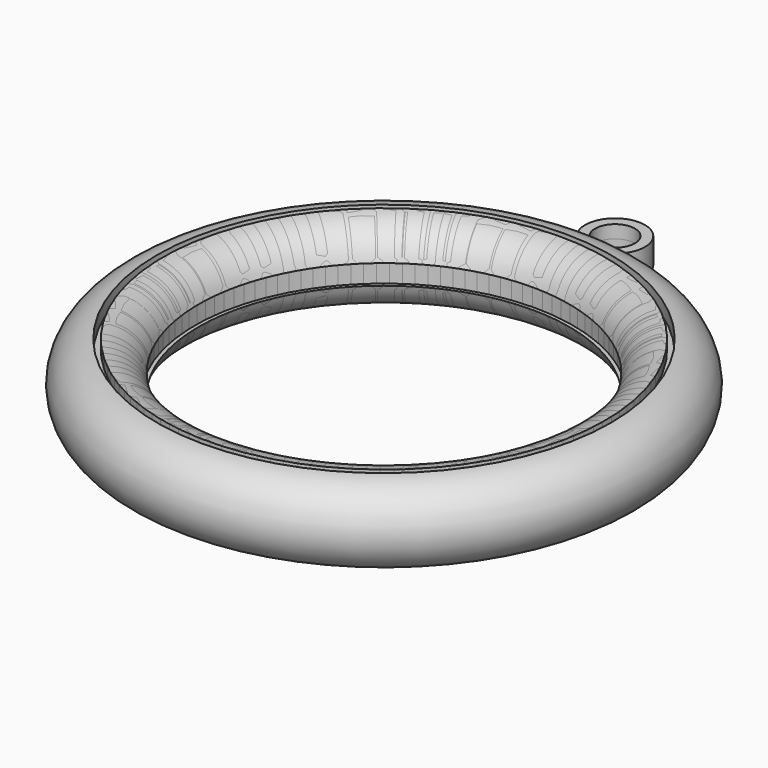
from build123d import *

# Parameters (mm, degrees)
F3_R          = 3
F3_R_2        = 2
F4_DEPTH      = 1.3
F4_DEPTH_BACK = 1.3
F1_R          = 1.5


with BuildPart() as f2:
    # F2: sweep along a path in F0
    with BuildLine(Plane.XY) as f2_path:
        CenterArc((0, 0), 22.5, 0, 360)
    # F1 (on Right) → F2 (sweep)
    with BuildSketch(Plane.YZ):
        with BuildLine():
            Line((22.2, 3.0352100422), (22.2, 3.988734135))
            ThreePointArc((22.2, 3.988734135), (19.9335665926, 3.0681296527), (18.6270166538, 1))
            Line((18.6270166538, 1), (19, 1))
            Line((19, 1), (19, -1))
            Line((19, -1), (18.6270166538, -1))
            ThreePointArc((18.6270166538, -1), (19.9335665926, -3.0681296527), (22.2, -3.988734135))
            Line((22.2, -3.988734135), (22.2, -3.0352100422))
            ThreePointArc((22.2, -3.0352100422), (19.45, 0), (22.2, 3.0352100422))
        make_face()
    sweep(path=f2_path.line)


with BuildPart() as f4:
    # F3 (on Top) → F4 (new body, two sides)
    with BuildSketch(Plane.XY) as f4_sk:
        with Locations((0, 29)):
            Circle(F3_R)
        with Locations((0, 29)):
            Circle(F3_R_2, mode=Mode.SUBTRACT)
    extrude(amount=F4_DEPTH)
    extrude(f4_sk.sketch, amount=-F4_DEPTH_BACK)

    # F1 (on Right) → F6, piece 2 (revolve)
    with BuildSketch(Plane.YZ):
        with BuildLine():
            Line((22.8, 3.988734135), (22.8, 2.6329641091))
            ThreePointArc((22.8, 2.6329641091), (19.85, 0), (22.8, -2.6329641091))
            Line((22.8, -2.6329641091), (22.8, -3.988734135))
            ThreePointArc((22.8, -3.988734135), (26.5, 0), (22.8, 3.988734135))
        make_face()
        with Locations((22.5, 0)):
            Circle(F1_R, mode=Mode.SUBTRACT)
    revolve(axis=Axis((0, 0, -12.8101566806), (0, 0, -1)))


with BuildPart() as f6:
    # F1 (on Right) → F6 (revolve)
    with BuildSketch(Plane.YZ):
        with BuildLine():
            Line((22.2, 3.0352100422), (22.2, 3.988734135))
            ThreePointArc((22.2, 3.988734135), (19.9335665926, 3.0681296527), (18.6270166538, 1))
            Line((18.6270166538, 1), (19, 1))
            Line((19, 1), (19, -1))
            Line((19, -1), (18.6270166538, -1))
            ThreePointArc((18.6270166538, -1), (19.9335665926, -3.0681296527), (22.2, -3.988734135))
            Line((22.2, -3.988734135), (22.2, -3.0352100422))
            ThreePointArc((22.2, -3.0352100422), (19.45, 0), (22.2, 3.0352100422))
        make_face()
    revolve(axis=Axis((0, 0, -12.8101566806), (0, 0, -1)))


solid = Compound([f2.part, f4.part, f6.part])
